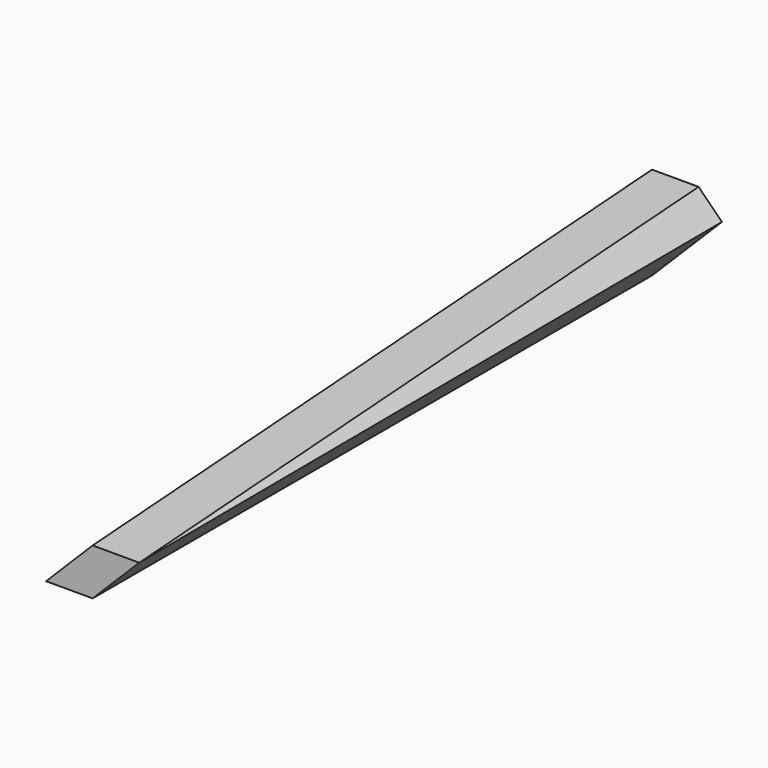
from build123d import *

# Parameters (mm, degrees)
F0_W        = 10.16
F0_H        = 5.08
F1_DEPTH    = 38.1
F2_SIZE2    = 2.53999
F2_SIZE     = 38.09999
F3_T1_DEPTH = 64.3128613158
F4_T1_DEPTH = 13.0641595789
F4_T3_DEPTH = 44.702137425
F5_T1_DEPTH = 64.1438766671


# Not quite as in the source:
# - a fillet or chamfer that OpenCascade refuses, or shapes differently, is made with other operations: its cross-section is extruded or revolved along the edge and cut away or added
# - a fillet or chamfer is up to 0.001 mm smaller than in the source, because OpenCascade refuses the exact size


with BuildPart() as f1:
    # F0 (on Front) → F1 (new body)
    with BuildSketch(Plane.XZ):
        with Locations((5.08, 2.54)):
            Rectangle(F0_W, F0_H)
    extrude(amount=F1_DEPTH)

    # F2 (size 38.1 and 2.54 in the source; OpenCascade refuses exactly that, so slightly less here)
    f2_edges = [f1.edges().sort_by_distance(p)[0] for p in [
        (5.08, -38.1, 5.08),
    ]]
    f2_side = f1.faces().sort_by_distance((5.08, -19.05, 5.08))[0]
    chamfer(f2_edges, length=F2_SIZE, length2=F2_SIZE2, reference=f2_side)

    # F3: chamfer of 5.08 on 1 edges, made by hand

    # F3_s2 → F3_t1 (cut)
    with BuildSketch(Plane(origin=(0, 13.3723717196, 0.8914881722), x_dir=(1, 0, 0), z_dir=(0, -0.9977851741, -0.0665187672))):
        Polygon((0, -0.0112506505), (5.08, 5.0687493495), (0, 5.0687493495), align=None)
    extrude(amount=F3_T1_DEPTH, mode=Mode.SUBTRACT)

    # F4: chamfer of 2.54 on 2 edges, made by hand

    # F4_s2 → F4_t1 (cut)
    with BuildSketch(Plane.XZ.offset(-6.5320747894)):
        Polygon((7.62, 5.08), (10.16, 2.54), (10.16, 5.08), align=None)
    extrude(amount=F4_T1_DEPTH, mode=Mode.SUBTRACT)

    # F4_s4 → F4_t3 (cut)
    with BuildSketch(Plane(origin=(0, 0.3226895493, 0.0215125576), x_dir=(1, 0, 0), z_dir=(0, -0.9977851741, -0.0665187672))):
        Polygon((7.62, 5.0687493495), (10.16, 2.5287493495), (10.16, 5.0687493495), align=None)
    extrude(amount=F4_T3_DEPTH, mode=Mode.SUBTRACT)

    # F5: chamfer of 5.08 on 1 edges, made by hand

    # F5_s2 → F5_t1 (cut)
    with BuildSketch(Plane.XZ.offset(-13.0641495789)):
        Polygon((10.16, 5.08), (5.08, 0), (10.16, 0), align=None)
    extrude(amount=F5_T1_DEPTH, mode=Mode.SUBTRACT)


solid = f1.part
